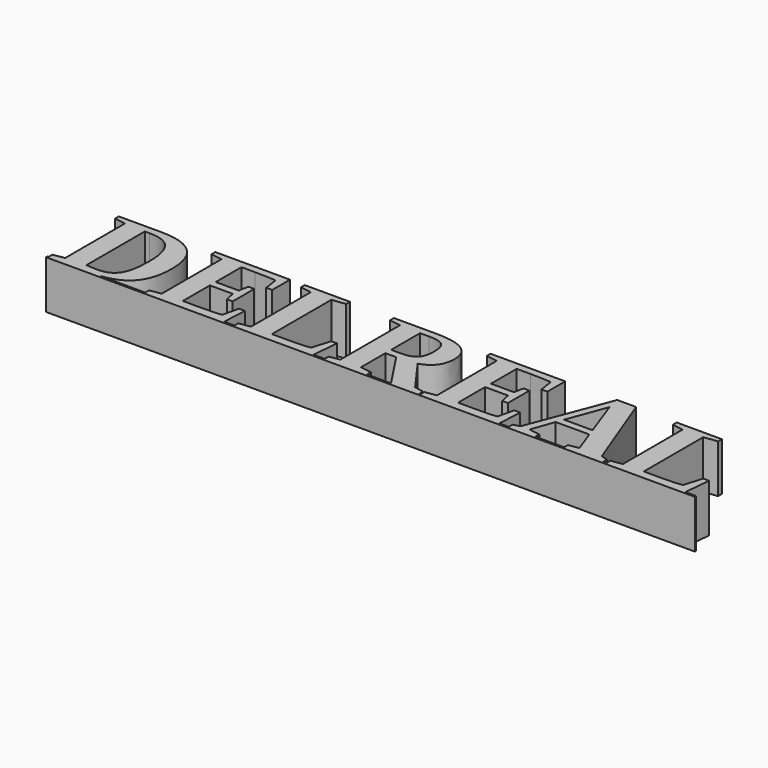
from build123d import *

# Parameters (mm, degrees)
F1_W         = 336.5535438061
F1_H         = 0.9047373314
F0_TEXT_SIZE = 69.4444444444
F2_DEPTH     = 25


# Not quite as in the source:
# - Text() gives the source's letters only with a copy of the font that has no kerning and outlines rounded to 1/6400 em; it was checked with that copy


with BuildPart() as f2:
    # F1 (on Top) + F0 (on Top) → F2 (new body)
    with BuildSketch(Plane.XY):
        with Locations((-168.276771903, -0.4523686657)):
            Rectangle(F1_W, F1_H)
    with BuildSketch(Plane.XY):
        with Locations((-337.1636284722, 0)):
            Text('DELREAL', F0_TEXT_SIZE, font='Tinos', font_style=FontStyle.BOLD, text_align=(TextAlign.LEFT, TextAlign.BOTTOM))
    extrude(amount=F2_DEPTH)


solid = f2.part
